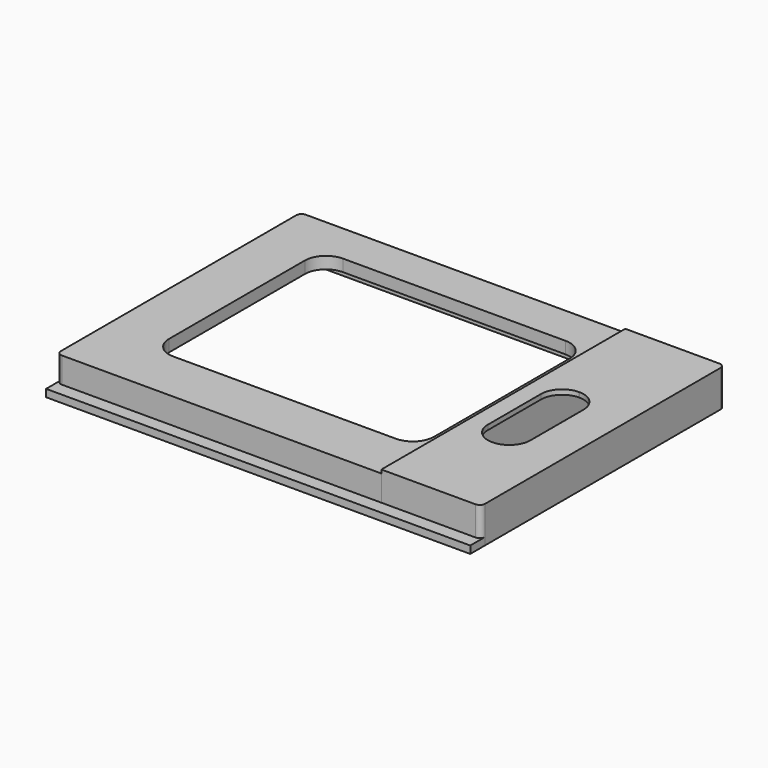
from build123d import *

# Parameters (mm, degrees)
F0_W     = 77.7997439444
F0_H     = 73.0322113484
F0_W_2   = 63.5
F0_H_2   = 50.8
F1_DEPTH = 7.9375
F0_W_3   = 23.8320640683
F0_W_4   = 10.1920276119
F0_H_3   = 26.0350044244
F2_DEPTH = 8.7757
F4_DEPTH = 5.08
F5_W     = 16.2187814713
F5_H     = 65.4515903443
F6_DEPTH = 7.62
F7_W     = 101.6318080127
F7_H     = 7.0125763357
F8_DEPTH = 1.778
F7_W_2   = 77.7997859359
F7_H_2   = 3.8491855323
F9_DEPTH = 1.778
F10_R    = 5.08
F11_R    = 5.08
F12_R    = 1.27
F12_2_R  = 1.27


# Not quite as in the source:
# - ends of sketch curves that miss each other by under 0.0002 mm in the source are joined
# - a feature names something its author has since deleted; it is built from what else it names


with BuildPart() as f1:
    # F0 (on Top) → F1 (new body)
    with BuildSketch(Plane.XY):
        with Locations((-5.5623719722, -1.5838943258)):
            Rectangle(F0_W, F0_H)
        Rectangle(F0_W_2, F0_H_2, mode=Mode.SUBTRACT)
    extrude(amount=F1_DEPTH)

    # F3 (on face) → F4 (cut)
    with BuildSketch(Plane.XY):
        Polygon((32.3214142647, 31.8624414504), (-40.6522077048, 31.8624414504), (-40.6522077048, -34.2938601971), (32.3214142647, -34.2938601971), (32.3214142647, 0), align=None)
    extrude(amount=F4_DEPTH, mode=Mode.SUBTRACT)


with BuildPart() as f2:
    # F0 (on Top) → F2 (new body)
    with BuildSketch(Plane.XY):
        with Locations((45.2535320342, -1.5838943258)):
            Rectangle(F0_W_3, F0_H)
        with Locations((42.6406442738, -3.4959255073)):
            Rectangle(F0_W_4, F0_H_3, mode=Mode.SUBTRACT)
    extrude(amount=F2_DEPTH)

    # F5 (on face) → F6 (cut)
    with BuildSketch(Plane.XY):
        with Locations((45.3053861856, -1.6035111621)):
            Rectangle(F5_W, F5_H)
    extrude(amount=F6_DEPTH, mode=Mode.SUBTRACT)


with BuildPart() as f8_tool:
    # F7 (on face) → F8 (new body)
    with BuildSketch(Plane.XY):
        with Locations((6.3536180705, -37.7571026355)):
            Rectangle(F7_W, F7_H)
    extrude(amount=F8_DEPTH)


with BuildPart() as f1_1:
    add(f1.part)

    # F8: cut by f8_tool
    add(f8_tool.part, mode=Mode.SUBTRACT)

    # F10
    f10_edges = [f1_1.edges().sort_by_distance(p)[0] for p in [
        (31.75, 25.4, 6.50875),
        (-31.75, 25.4, 6.50875),
        (31.75, -25.4, 6.50875),
        (-31.75, -25.4, 6.50875),
    ]]
    fillet(f10_edges, radius=F10_R)

    # F12
    f12_edges = [f1_1.edges().sort_by_distance(p)[0] for p in [
        (-44.462244, 34.932211, 3.96875),
        (-44.462244, -38.1, 4.85775),
    ]]
    fillet(f12_edges, radius=F12_R)


with BuildPart() as f2_1:
    add(f2.part)

    # F8: cut by f8_tool
    add(f8_tool.part, mode=Mode.SUBTRACT)

    # F11
    f11_edges = [f2_1.edges().sort_by_distance(p)[0] for p in [
        (47.736658, 9.521577, 8.19785),
        (47.736658, -16.513428, 8.19785),
        (37.54463, -16.513428, 8.19785),
        (37.54463, 9.521577, 8.19785),
    ]]
    fillet(f11_edges, radius=F11_R)

    # F12#2
    f12_2_edges = [f2_1.edges().sort_by_distance(p)[0] for p in [
        (57.169564, 34.932211, 4.38785),
        (57.169564, -38.1, 4.38785),
    ]]
    fillet(f12_2_edges, radius=F12_2_R)


with BuildPart() as f9:
    # F7 (on face) → F9 (new body)
    with BuildSketch(Plane.XY):
        Polygon((-44.4622859359, -38.1), (-44.4622859359, -41.2633908033), (57.1695220768, -41.2633908033), (57.1695220768, -34.2508144677), (33.3375, -34.2508144677), (33.3375, -38.1), align=None)
        with Locations((-5.5623929679, -36.1754072338)):
            Rectangle(F7_W_2, F7_H_2)
    extrude(amount=F9_DEPTH)


solid = Compound([f1_1.part, f2_1.part, f9.part])
